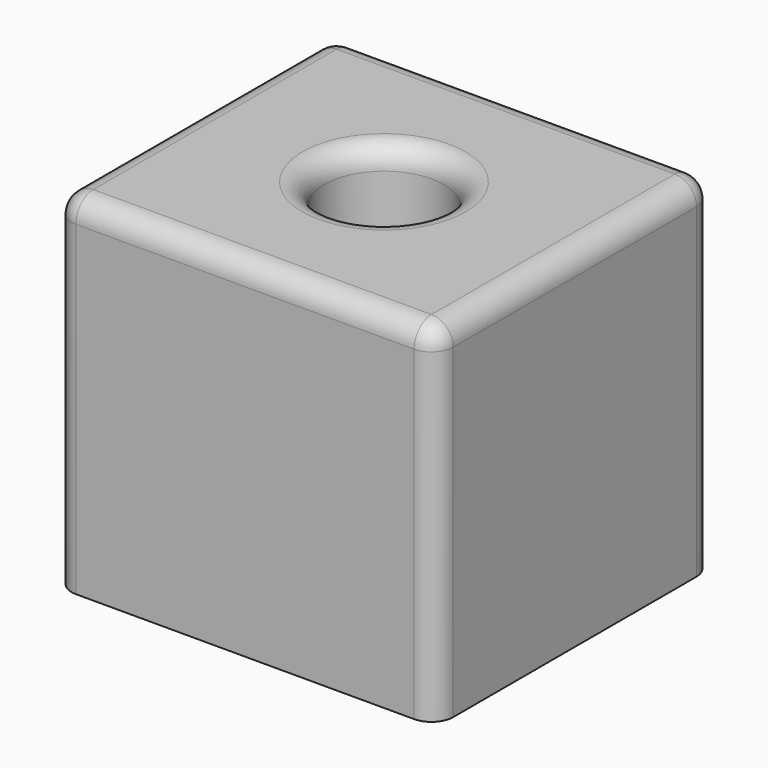
from build123d import *

# Parameters (mm, degrees)
F0_W          = 87.8805932263
F0_H          = 80
F1_DEPTH      = 80
F2_R          = 13.7808794965
F3_DEPTH      = 25
F4_R          = 13.7808794965
F7_DEPTH      = 25
F5_R          = 13.7808794965
F8_DEPTH      = 25
F6_R          = 13.7808794965
F9_DEPTH      = 105.001
F10_R         = 5
F11_T1_DEPTH  = 87.5
F11_S5_W      = 5
F11_S5_H      = 5
F11_T6_DEPTH  = 5
F11_S11_W     = 5
F11_S11_H     = 5
F11_T12_DEPTH = 5
F11_S17_W     = 5
F11_S17_H     = 5
F11_T18_DEPTH = 5
F11_S23_W     = 5
F11_S23_H     = 5
F11_T24_DEPTH = 5


# Not quite as in the source:
# - a fillet or chamfer that OpenCascade refuses, or shapes differently, is made with other operations: its cross-section is extruded or revolved along the edge and cut away or added


with BuildPart() as f1:
    # F0 (on Top) → F1 (new body)
    with BuildSketch(Plane.XY):
        Rectangle(F0_W, F0_H)
    extrude(amount=F1_DEPTH)

    # F2 (on face) → F3 (join)
    with BuildSketch(Plane.XY.offset(80)):
        Circle(F2_R)
    extrude(amount=F3_DEPTH)

    # F4 (on face) → F7 (cut)
    with BuildSketch(Plane.XY.offset(105)):
        Circle(F4_R)
    extrude(amount=-F7_DEPTH, mode=Mode.SUBTRACT)

    # F5 (on face) → F8 (cut)
    with BuildSketch(Plane.XY):
        Circle(F5_R)
    extrude(amount=-F8_DEPTH, mode=Mode.SUBTRACT)

    # F6 (on face) → F9 (cut, through all)
    with BuildSketch(Plane.XY.offset(105)):
        Circle(F6_R)
    extrude(amount=-F9_DEPTH, mode=Mode.SUBTRACT)

    # F10
    f10_edges = [f1.edges().sort_by_distance(p)[0] for p in [
        (0, 40, 80),
        (43.940297, 0, 80),
        (-43.940297, 0, 80),
        (0, -40, 80),
        (-13.780879, 0, 80),
    ]]
    fillet(f10_edges, radius=F10_R)

    # F11: fillet of radius 5 on 15 edges, made by hand

    # F11_s2 → F11_t1 (cut)
    with BuildSketch(Plane.XY.offset(-12.5)):
        with BuildLine():
            ThreePointArc((-43.9402966131, -35), (-42.4758305191, -38.5355339059), (-38.9402966131, -40))
            Line((-38.9402966131, -40), (-43.9402966131, -40))
            Line((-43.9402966131, -40), (-43.9402966131, -35))
        make_face()
        with BuildLine():
            ThreePointArc((43.9402966131, -35), (42.4758305191, -38.5355339059), (38.9402966131, -40))
            Line((38.9402966131, -40), (43.9402966131, -40))
            Line((43.9402966131, -40), (43.9402966131, -35))
        make_face()
        with BuildLine():
            ThreePointArc((-38.9402966131, 40), (-42.4758305191, 38.5355339059), (-43.9402966131, 35))
            Line((-43.9402966131, 35), (-43.9402966131, 40))
            Line((-43.9402966131, 40), (-38.9402966131, 40))
        make_face()
        with BuildLine():
            ThreePointArc((38.9402966131, 40), (42.4758305191, 38.5355339059), (43.9402966131, 35))
            Line((43.9402966131, 35), (43.9402966131, 40))
            Line((43.9402966131, 40), (38.9402966131, 40))
        make_face()
    extrude(amount=F11_T1_DEPTH, mode=Mode.SUBTRACT)


with BuildPart() as f11_tool4:
    # F11_s5 → F11_t6 (new body)
    with BuildSketch(Plane.XZ.offset(-35)):
        with Locations((41.4402966131, 77.5)):
            Rectangle(F11_S5_W, F11_S5_H)
    extrude(amount=-F11_T6_DEPTH)

    # F11_s7 → F11_t8 (revolve, cut)
    with BuildSketch(Plane(origin=(38.9402966131, 35, 75), x_dir=(-0.7071067812, 0, -0.7071067812), z_dir=(0.7071067812, 0, -0.7071067812))):
        with BuildLine():
            ThreePointArc((0, -5), (5, 0), (0, 5))
            Line((0, 5), (0, -5))
        make_face()
    revolve(axis=Axis((38.9402966131, 35, 75), (0, 1, 0)), mode=Mode.SUBTRACT)


with BuildPart() as f1_1:
    add(f1.part)

    # F11_t3: cut F11_tool4
    add(f11_tool4.part, mode=Mode.SUBTRACT)


with BuildPart() as f11_tool10:
    # F11_s11 → F11_t12 (new body)
    with BuildSketch(Plane.XZ.offset(-35)):
        with Locations((-41.4402966131, 77.5)):
            Rectangle(F11_S11_W, F11_S11_H)
    extrude(amount=-F11_T12_DEPTH)

    # F11_s13 → F11_t14 (revolve, cut)
    with BuildSketch(Plane(origin=(-38.9402966131, 35, 75), x_dir=(0.7071067812, 0, -0.7071067812), z_dir=(0.7071067812, 0, 0.7071067812))):
        with BuildLine():
            ThreePointArc((0, -5), (5, 0), (0, 5))
            Line((0, 5), (0, -5))
        make_face()
    revolve(axis=Axis((-38.9402966131, 35, 75), (0, 1, 0)), mode=Mode.SUBTRACT)


with BuildPart() as f1_2:
    add(f1_1.part)

    # F11_t9: cut F11_tool10
    add(f11_tool10.part, mode=Mode.SUBTRACT)


with BuildPart() as f11_tool16:
    # F11_s17 → F11_t18 (new body)
    with BuildSketch(Plane.YZ.offset(38.9402966131)):
        with Locations((-37.5, 77.5)):
            Rectangle(F11_S17_W, F11_S17_H)
    extrude(amount=F11_T18_DEPTH)

    # F11_s19 → F11_t20 (revolve, cut)
    with BuildSketch(Plane(origin=(38.9402966131, -35, 75), x_dir=(0, 0.7071067812, -0.7071067812), z_dir=(0, -0.7071067812, -0.7071067812))):
        with BuildLine():
            ThreePointArc((0, -5), (5, 0), (0, 5))
            Line((0, 5), (0, -5))
        make_face()
    revolve(axis=Axis((38.9402966131, -35, 75), (1, 0, 0)), mode=Mode.SUBTRACT)


with BuildPart() as f1_3:
    add(f1_2.part)

    # F11_t15: cut F11_tool16
    add(f11_tool16.part, mode=Mode.SUBTRACT)


with BuildPart() as f11_tool22:
    # F11_s23 → F11_t24 (new body)
    with BuildSketch(Plane.YZ.offset(-38.9402966131)):
        with Locations((-37.5, 77.5)):
            Rectangle(F11_S23_W, F11_S23_H)
    extrude(amount=-F11_T24_DEPTH)

    # F11_s25 → F11_t26 (revolve, cut)
    with BuildSketch(Plane(origin=(-38.9402966131, -35, 75), x_dir=(0, 0.7071067812, -0.7071067812), z_dir=(0, 0.7071067812, 0.7071067812))):
        with BuildLine():
            ThreePointArc((0, -5), (5, 0), (0, 5))
            Line((0, 5), (0, -5))
        make_face()
    revolve(axis=Axis((-38.9402966131, -35, 75), (-1, 0, 0)), mode=Mode.SUBTRACT)


with BuildPart() as f1_4:
    add(f1_3.part)

    # F11_t21: cut F11_tool22
    add(f11_tool22.part, mode=Mode.SUBTRACT)


solid = f1_4.part
